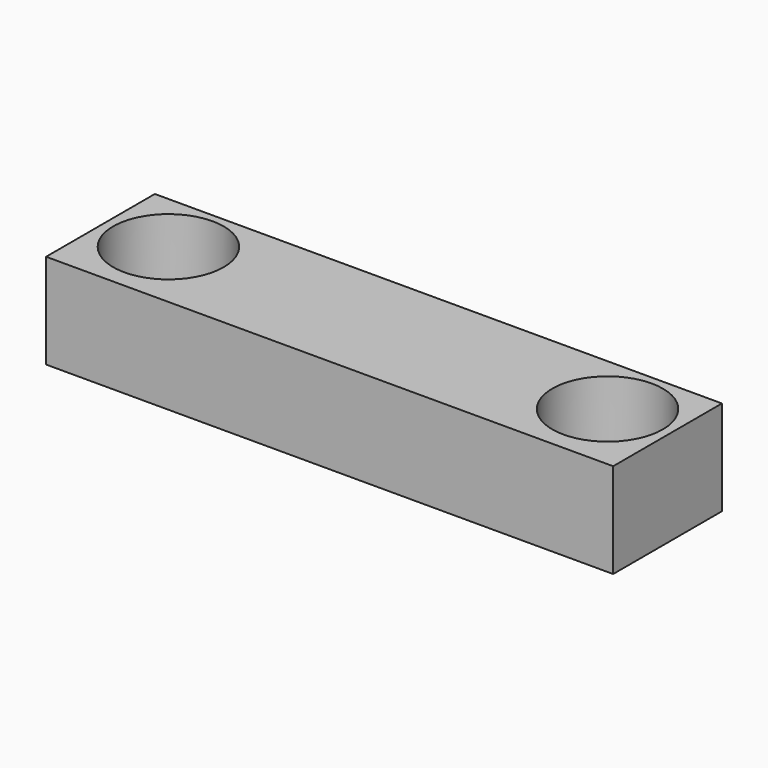
from build123d import *

# Parameters (mm, degrees)
F0_W     = 151.7232432961
F0_H     = 36.3720078021
F0_R     = 14.7880803575
F1_DEPTH = 25.4


# Not quite as in the source:
# - a feature names something its author has since deleted; it is built from what else it names


with BuildPart() as f1:
    # F0 (on Top) → F1 (new body)
    with BuildSketch(Plane.XY):
        with Locations((-0.0307895243, 41.7389301583)):
            Rectangle(F0_W, F0_H)
        with Locations((-58.7456077337, 43.0379323661)):
            Circle(F0_R, mode=Mode.SUBTRACT)
        with Locations((58.7456077337, 43.0379323661)):
            Circle(F0_R, mode=Mode.SUBTRACT)
    extrude(amount=F1_DEPTH)


solid = f1.part
